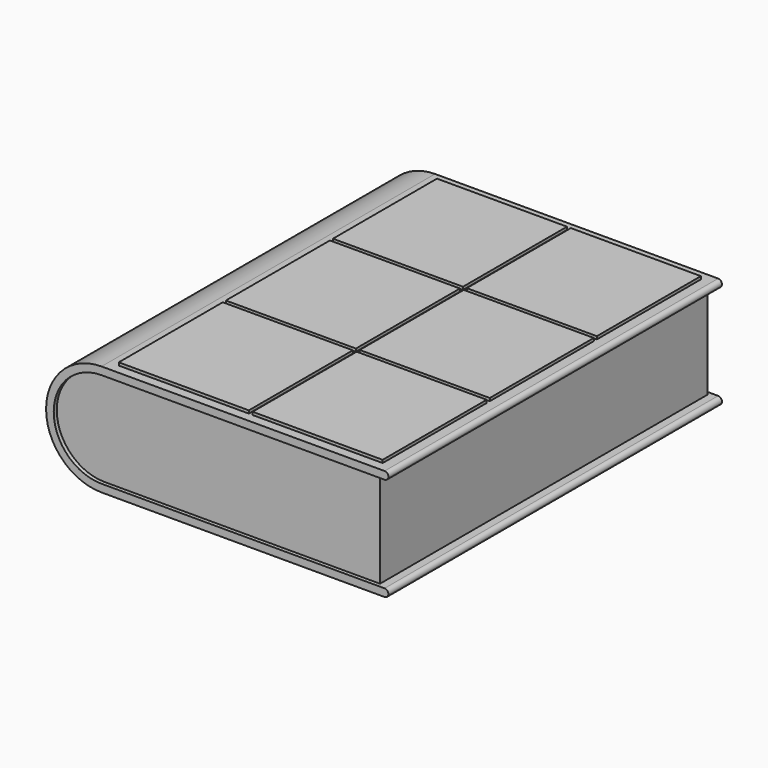
from build123d import *

# Parameters (mm, degrees)
F1_DEPTH = 109
F3_DEPTH = 107
F4_W     = 68
F4_H     = 68
F5_DEPTH = 1.5


# Not quite as in the source:
# - ends of sketch curves that miss each other by under 0.0002 mm in the source are joined


with BuildPart() as f1:
    # F0 (on Front) → F1 (new body, symmetric)
    with BuildSketch(Plane.XZ):
        with BuildLine():
            ThreePointArc((0, -25), (-25, 0), (0, 25))
            Line((0, 25), (148, 25))
            ThreePointArc((148, 25), (150, 26.9999995828), (148, 28.9999995828))
            Line((148, 28.9999995828), (0, 28.9999991655))
            ThreePointArc((0, 28.9999991655), (-28.9999991655, 0), (0, -28.9999991655))
            Line((0, -28.9999991655), (148, -28.9999991655))
            ThreePointArc((148, -28.9999991655), (150, -26.9999995828), (148, -24.9999995828))
            Line((148, -24.9999995828), (0, -25))
        make_face()
    extrude(amount=F1_DEPTH, both=True)

    # F2 (on Front) → F3 (join, symmetric)
    with BuildSketch(Plane.XZ):
        with BuildLine():
            Line((144, 25), (0, 25))
            ThreePointArc((0, 25), (-25, 0), (0, -25))
            Line((0, -25), (144, -25))
            Line((144, -25), (144, 25))
        make_face()
    extrude(amount=F3_DEPTH, both=True)

    # F4 (on face) → F5 (join)
    with BuildSketch(Plane.XY.offset(28.9999991655)):
        with Locations((39, 70)):
            Rectangle(F4_W, F4_H)
        with Locations((39, 0)):
            Rectangle(F4_W, F4_H)
        with Locations((39, -70)):
            Rectangle(F4_W, F4_H)
        with Locations((109, 70)):
            Rectangle(F4_W, F4_H)
        with Locations((109, 0)):
            Rectangle(F4_W, F4_H)
        with Locations((109, -70)):
            Rectangle(F4_W, F4_H)
    extrude(amount=F5_DEPTH)


solid = f1.part
